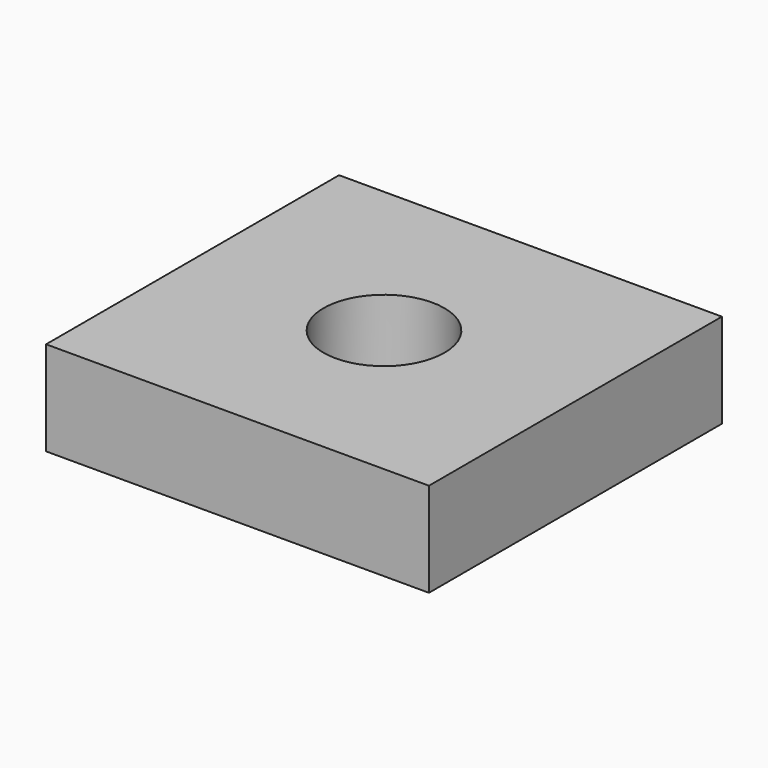
from build123d import *

# Parameters (mm, degrees)
F0_R     = 16.2815755653
F1_DEPTH = 25.4
F3_DEPTH = 25.4


# Not quite as in the source:
# - the program builds the solid bodies; features that only make, move or delete a surface that nothing else refers to are left out


with BuildPart() as f1:
    # F0 (on Top) → F1 (new body)
    with BuildSketch(Plane.XY):
        Polygon((-32.1844741702, 49.3294708431), (-51.5748507939, 49.3294708431), (-51.5748507939, -49.3294708431), (51.5748507939, -49.3294708431), (51.5748507939, 49.3294708431), (-11.7852937953, 49.3294708431), align=None)
        Circle(F0_R, mode=Mode.SUBTRACT)
    extrude(amount=F1_DEPTH)

    # F0 (on Top) → F3 (join)
    with BuildSketch(Plane.XY):
        Polygon((-32.1844741702, 49.3294708431), (-51.5748507939, 49.3294708431), (-51.5748507939, -49.3294708431), (51.5748507939, -49.3294708431), (51.5748507939, 49.3294708431), (-11.7852937953, 49.3294708431), align=None)
        Circle(F0_R, mode=Mode.SUBTRACT)
    extrude(amount=F3_DEPTH)


solid = f1.part
